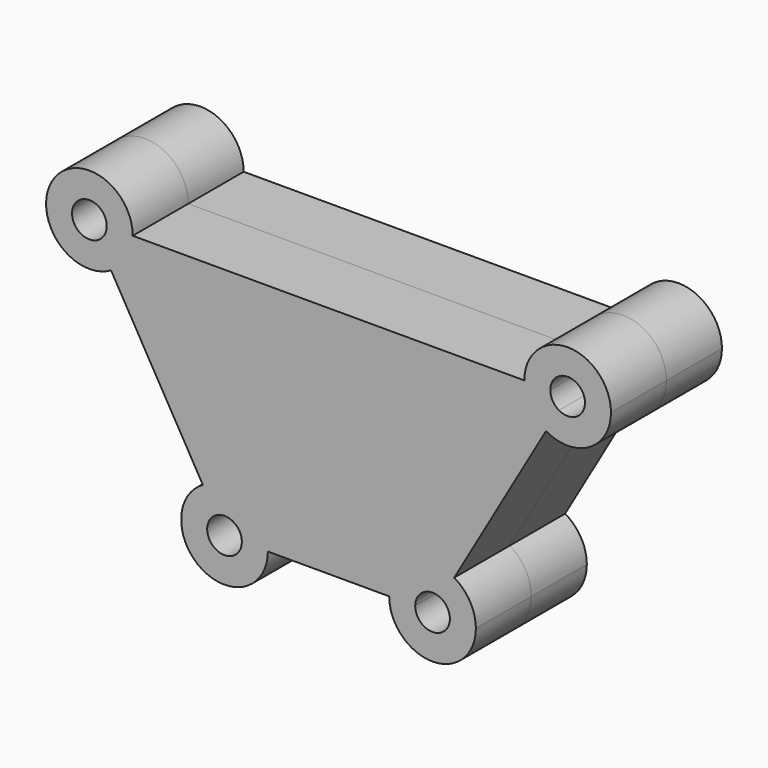
from build123d import *

# Parameters (mm, degrees)
F1_DEPTH = 50.8


with BuildPart() as f1:
    # F0 (on Front) → F1 (new body, symmetric)
    with BuildSketch(Plane.XZ):
        with BuildLine():
            ThreePointArc((-79.9545346996, -72.4959198801), (-67.2545346996, -72.4959198801), (-60.9045346996, -83.4944425082))
            Line((-60.9045346996, -83.4944425082), (-41.8545346996, -83.4944425082))
            ThreePointArc((-41.8545346996, -83.4944425082), (-57.7295346996, -55.998135938), (-89.4795346996, -55.998135938))
            Line((-89.4795346996, -55.998135938), (-79.9545346996, -72.4959198801))
        make_face()
        with BuildLine():
            Line((-41.8545346996, -83.4944425082), (-60.9045346996, -83.4944425082))
            ThreePointArc((-60.9045346996, -83.4944425082), (-79.9545346996, -94.4929651363), (-79.9545346996, -72.4959198801))
            Line((-79.9545346996, -72.4959198801), (-89.4795346996, -55.998135938))
            ThreePointArc((-89.4795346996, -55.998135938), (-89.4795346996, -110.9907490783), (-41.8545346996, -83.4944425082))
        make_face()
        with BuildLine():
            ThreePointArc((-89.4795346996, -55.998135938), (-57.7295346996, -55.998135938), (-41.8545346996, -83.4944425082))
            Line((-41.8545346996, -83.4944425082), (47.0454653004, -83.4944425082))
            ThreePointArc((47.0454653004, -83.4944425082), (62.9204653004, -55.998135938), (94.6704653004, -55.998135938))
            Line((94.6704653004, -55.998135938), (161.9071689529, 60.4592509217))
            ThreePointArc((161.9071689529, 60.4592509217), (150.2858623828, 72.0805574918), (146.0321689529, 87.9555574918))
            Line((146.0321689529, 87.9555574918), (-140.8412383522, 87.9555574918))
            ThreePointArc((-140.8412383522, 87.9555574918), (-145.094931782, 72.0805574918), (-156.7162383522, 60.4592509217))
            Line((-156.7162383522, 60.4592509217), (-89.4795346996, -55.998135938))
        make_face()
        with BuildLine():
            ThreePointArc((94.6704653004, -55.998135938), (62.9204653004, -55.998135938), (47.0454653004, -83.4944425082))
            Line((47.0454653004, -83.4944425082), (66.0954653004, -83.4944425082))
            ThreePointArc((66.0954653004, -83.4944425082), (72.4454653004, -72.4959198801), (85.1454653004, -72.4959198801))
            Line((85.1454653004, -72.4959198801), (94.6704653004, -55.998135938))
        make_face()
        with BuildLine():
            Line((66.0954653004, -83.4944425082), (47.0454653004, -83.4944425082))
            ThreePointArc((47.0454653004, -83.4944425082), (78.7954653004, -115.2444425082), (110.5454653004, -83.4944425082))
            ThreePointArc((110.5454653004, -83.4944425082), (106.2917718705, -67.6194425082), (94.6704653004, -55.998135938))
            Line((94.6704653004, -55.998135938), (85.1454653004, -72.4959198801))
            ThreePointArc((85.1454653004, -72.4959198801), (89.7939879284, -77.1444425082), (91.4954653004, -83.4944425082))
            ThreePointArc((91.4954653004, -83.4944425082), (78.7954653004, -96.1944425082), (66.0954653004, -83.4944425082))
        make_face()
        with BuildLine():
            ThreePointArc((-140.8412383522, 87.9555574918), (-200.0875449223, 103.8305574918), (-156.7162383522, 60.4592509217))
            Line((-156.7162383522, 60.4592509217), (-166.2412383522, 76.9570348637))
            ThreePointArc((-166.2412383522, 76.9570348637), (-183.5897609803, 94.3055574918), (-159.8912383522, 87.9555574918))
            Line((-159.8912383522, 87.9555574918), (-140.8412383522, 87.9555574918))
        make_face()
        with BuildLine():
            Line((-166.2412383522, 76.9570348637), (-156.7162383522, 60.4592509217))
            ThreePointArc((-156.7162383522, 60.4592509217), (-145.094931782, 72.0805574918), (-140.8412383522, 87.9555574918))
            Line((-140.8412383522, 87.9555574918), (-159.8912383522, 87.9555574918))
            ThreePointArc((-159.8912383522, 87.9555574918), (-161.5927157241, 81.6055574918), (-166.2412383522, 76.9570348637))
        make_face()
        with BuildLine():
            ThreePointArc((146.0321689529, 87.9555574918), (150.2858623828, 72.0805574918), (161.9071689529, 60.4592509217))
            Line((161.9071689529, 60.4592509217), (171.4321689529, 76.9570348637))
            ThreePointArc((171.4321689529, 76.9570348637), (166.7836463249, 81.6055574918), (165.0821689529, 87.9555574918))
            Line((165.0821689529, 87.9555574918), (146.0321689529, 87.9555574918))
        make_face()
        with BuildLine():
            Line((171.4321689529, 76.9570348637), (161.9071689529, 60.4592509217))
            ThreePointArc((161.9071689529, 60.4592509217), (193.6571689529, 60.4592509217), (209.5321689529, 87.9555574918))
            ThreePointArc((209.5321689529, 87.9555574918), (177.7821689529, 119.7055574918), (146.0321689529, 87.9555574918))
            Line((146.0321689529, 87.9555574918), (165.0821689529, 87.9555574918))
            ThreePointArc((165.0821689529, 87.9555574918), (177.7821689529, 100.6555574918), (190.4821689529, 87.9555574918))
            ThreePointArc((190.4821689529, 87.9555574918), (184.1321689529, 76.9570348637), (171.4321689529, 76.9570348637))
        make_face()
    extrude(amount=F1_DEPTH, both=True)


solid = f1.part
